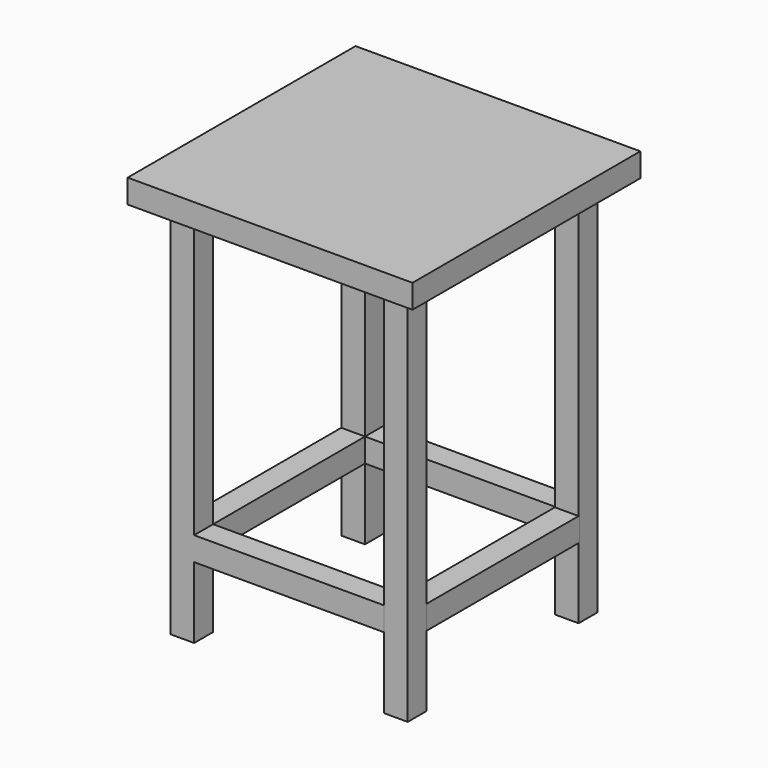
from build123d import *

# Parameters (mm, degrees)
F0_W      = 60
F0_H      = 60
F1_DEPTH  = 5
F3_W      = 5
F3_H      = 5
F4_DEPTH  = 80
F5_DEPTH  = 80
F6_DEPTH  = 80
F7_W      = 5
F7_H      = 5.0002082646
F8_DEPTH  = 40.1
F9_W      = 5
F9_H      = 5
F10_DEPTH = 40.2
F11_W     = 5
F11_H     = 5
F12_DEPTH = 40.2
F13_W     = 5
F13_H     = 5
F14_DEPTH = 40.2


with BuildPart() as f1:
    # F0 (on Top) → F1 (new body)
    with BuildSketch(Plane.XY):
        with Locations((-0.6647109985, -1.4024986219)):
            Rectangle(F0_W, F0_H)
    extrude(amount=F1_DEPTH)


with BuildPart() as f4:
    # F3 (on offset) → F4 (new body)
    with BuildSketch(Plane.XY.offset(-0.1)):
        with Locations((-23.1647109985, -23.9024986219)):
            Rectangle(F3_W, F3_H)
    extrude(amount=-F4_DEPTH)

    # F7 (on face) → F8 (join)
    with BuildSketch(Plane.YZ.offset(-20.6647109985)):
        with Locations((-23.9024986219, -62.5998958677)):
            Rectangle(F7_W, F7_H)
    extrude(amount=F8_DEPTH)


with BuildPart() as f5:
    # F3 (on offset) → F5 (new body)
    with BuildSketch(Plane.XY.offset(-0.1)):
        with Locations((21.8352890015, -23.9024986219)):
            Rectangle(F3_W, F3_H)
    extrude(amount=-F5_DEPTH)


with BuildPart() as f6:
    # F3 (on offset) → F6 (new body)
    with BuildSketch(Plane.XY.offset(-0.1)):
        with Locations((21.8352890015, 21.0975013781)):
            Rectangle(F3_W, F3_H)
    extrude(amount=-F6_DEPTH)


with BuildPart() as f6b:
    # F3 (on offset) → F6, piece 2 (new body)
    with BuildSketch(Plane.XY.offset(-0.1)):
        with Locations((-23.1647109985, 21.0975013781)):
            Rectangle(F3_W, F3_H)
    extrude(amount=-F6_DEPTH)


with BuildPart() as f10:
    # F9 (on face) → F10 (new body)
    with BuildSketch(Plane(origin=(0, -21.4024986219, 0), x_dir=(-1, 0, 0), z_dir=(0, 1, 0))):
        with Locations((-21.8352890015, -62.712443471)):
            Rectangle(F9_W, F9_H)
    extrude(amount=F10_DEPTH)


with BuildPart() as f12:
    # F11 (on face) → F12 (new body)
    with BuildSketch(Plane(origin=(19.3352890015, 0, 0), x_dir=(0, -1, 0), z_dir=(-1, 0, 0))):
        with Locations((-21.0975013781, -62.6)):
            Rectangle(F11_W, F11_H)
    extrude(amount=F12_DEPTH)


with BuildPart() as f14:
    # F13 (on face) → F14 (new body)
    with BuildSketch(Plane.XZ.offset(-18.5975013781)):
        with Locations((-23.1647109985, -62.6)):
            Rectangle(F13_W, F13_H)
    extrude(amount=F14_DEPTH)


solid = Compound([f1.part, f4.part, f5.part, f6.part, f6b.part, f10.part, f12.part, f14.part])
